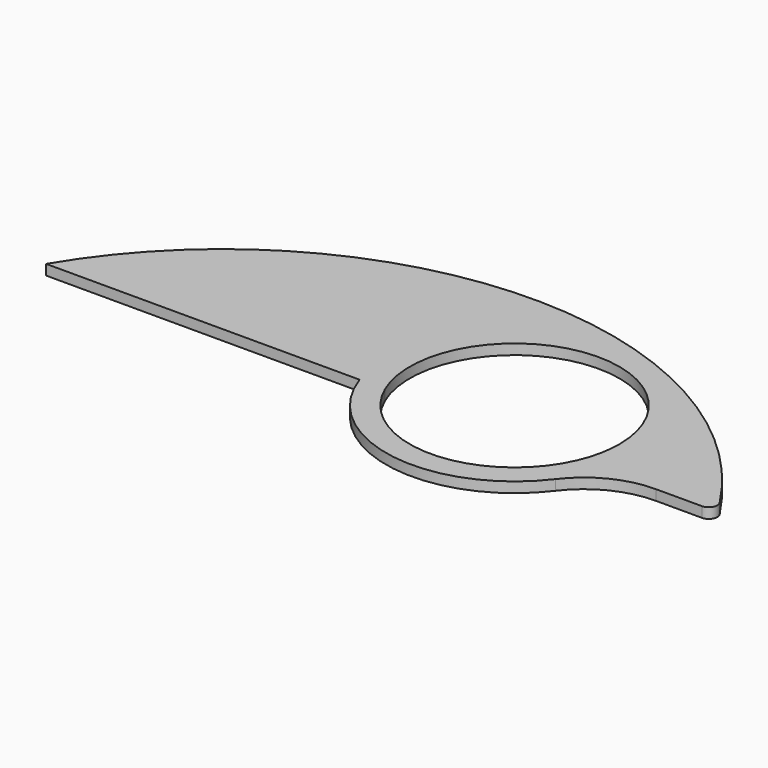
from build123d import *

# Parameters (mm, degrees)
F0_R      = 27.305
F1_DEPTH  = 0.8382
F3_DEPTH  = 25.4
F5_DEPTH  = 25.4
F9_DEPTH  = 0.8382
F10_DEPTH = 17.5768
F11_R     = 7.312924092
F12_R     = 0.6966323576


with BuildPart() as f1:
    # F0 (on Top) → F1 (new body)
    with BuildSketch(Plane.XY):
        Circle(F0_R)
    extrude(amount=F1_DEPTH)

    # F2 (on face) → F3 (cut)
    with BuildSketch(Plane.XY.offset(0.8382)):
        with BuildLine():
            Line((27.305, 0), (-27.305, 0))
            ThreePointArc((-27.305, 0), (0, -27.305), (27.305, 0))
        make_face()
    extrude(amount=-F3_DEPTH, mode=Mode.SUBTRACT)

    # F4 (on face) → F5 (cut)
    with BuildSketch(Plane.XY.offset(0.8382)):
        with BuildLine():
            ThreePointArc((-27.305, 0), (0, 15.5481644558), (27.305, 0))
            ThreePointArc((27.305, 0), (0, 27.305), (-27.305, 0))
        make_face()
    extrude(amount=-F5_DEPTH, mode=Mode.SUBTRACT)

    # F7 (on face) + F6 (on face) → F9 (join)
    with BuildSketch(Plane.XY.offset(0.8382)):
        with BuildLine():
            Line((-1.7974979465, 0), (18.003700975, 0))
            ThreePointArc((18.003700975, 0), (18.4250061935, 1.6697896776), (18.566720813, 3.3860683907))
            ThreePointArc((18.566720813, 3.3860683907), (6.3868228012, 13.7079730699), (-1.7974979465, 0))
        make_face()
    with BuildSketch(Plane.XY.offset(0.8382)):
        with BuildLine():
            Line((18.003700975, 0), (-1.7974979465, 0))
            ThreePointArc((-1.7974979465, 0), (8.1031015143, -7.077550908), (18.003700975, 0))
        make_face()
    extrude(amount=-F9_DEPTH)

    # F8 (on face) → F10 (cut)
    with BuildSketch(Plane.XY.offset(0.8382)):
        with BuildLine():
            ThreePointArc((15.935749386, 0), (16.4593427121, 1.6571771644), (16.6363208264, 3.3860683907))
            ThreePointArc((16.6363208264, 3.3860683907), (6.374210288, 11.7423095885), (0.2704536426, 0))
            Line((0.2704536426, 0), (15.935749386, 0))
        make_face()
        with BuildLine():
            Line((15.935749386, 0), (0.2704536426, 0))
            ThreePointArc((0.2704536426, 0), (8.1031015143, -5.1471509214), (15.935749386, 0))
        make_face()
    extrude(amount=-F10_DEPTH, mode=Mode.SUBTRACT)

    # F11
    f11_edges = [f1.edges().sort_by_distance(p)[0] for p in [
        (18.003701, 0, 0.4191),
    ]]
    fillet(f11_edges, radius=F11_R)

    # F12
    f12_edges = [f1.edges().sort_by_distance(p)[0] for p in [
        (27.305, 0, 0.4191),
    ]]
    fillet(f12_edges, radius=F12_R)


solid = f1.part
